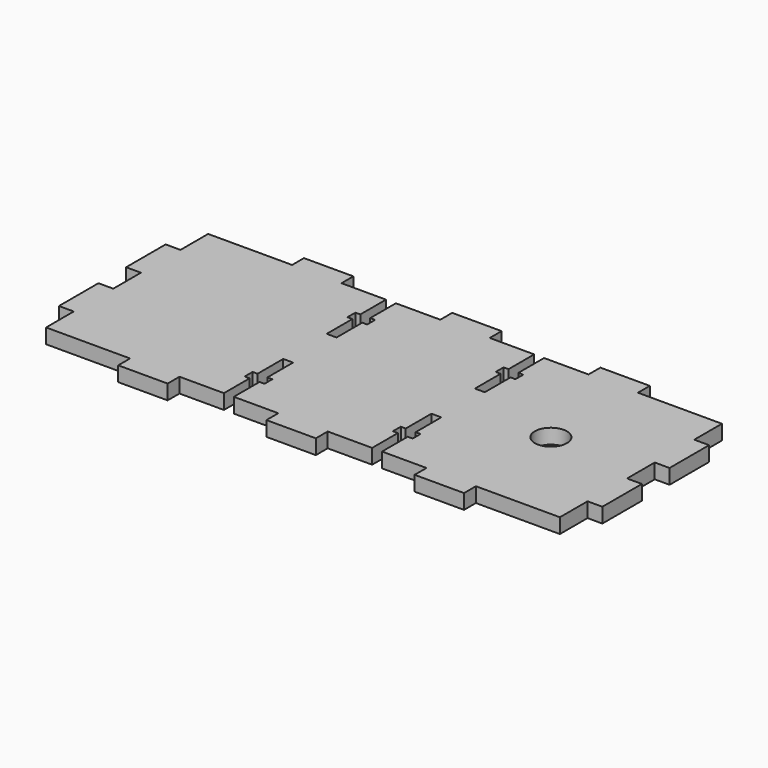
from build123d import *

# Parameters (mm, degrees)
F0_R     = 3.25
F1_DEPTH = 3


# Not quite as in the source:
# - a feature names something its author has since deleted; it is built from what else it names


with BuildPart() as f1:
    # F0 (on Top) → F1 (new body)
    with BuildSketch(Plane.XY):
        Polygon((0, 7), (0, 0), (17, 0), (17, -3), (27, -3), (27, 0), (36, 0), (36, 6.5), (35, 6.5), (35, 8.5), (36, 8.5), (36, 15), (38, 15), (38, 8.5), (39, 8.5), (39, 6.5), (38, 6.5), (38, 0), (47, 0), (47, -3), (57, -3), (57, 0), (66, 0), (66, 6.5), (65, 6.5), (65, 8.5), (66, 8.5), (66, 15), (68, 15), (68, 8.5), (69, 8.5), (69, 6.5), (68, 6.5), (68, 0), (77, 0), (77, -3), (87, -3), (87, 0), (104, 0), (104, 7), (107, 7), (107, 17), (104, 17), (104, 24), (107, 24), (107, 34), (104, 34), (104, 41), (87, 41), (87, 44), (77, 44), (77, 41), (68, 41), (68, 34.5), (69, 34.5), (69, 32.5), (68, 32.5), (68, 26), (66, 26), (66, 32.5), (65, 32.5), (65, 34.5), (66, 34.5), (66, 41), (57, 41), (57, 44), (47, 44), (47, 41), (38, 41), (38, 34.5), (39, 34.5), (39, 32.5), (38, 32.5), (38, 26), (36, 26), (36, 32.5), (35, 32.5), (35, 34.5), (36, 34.5), (36, 41), (27, 41), (27, 44), (17, 44), (17, 41), (0, 41), (0, 34), (-3, 34), (-3, 24), (0, 24), (0, 17), (-3, 17), (-3, 7), align=None)
        with Locations((85.7752785087, 20.5)):
            Circle(F0_R, mode=Mode.SUBTRACT)
    extrude(amount=F1_DEPTH)


solid = f1.part
